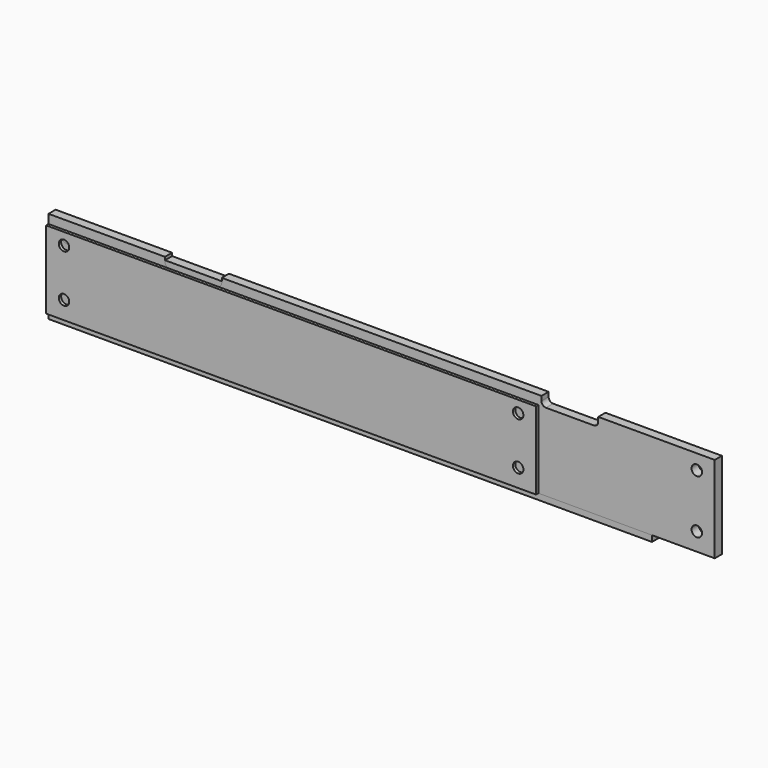
from build123d import *

# Parameters (mm, degrees)
F31_DEPTH       = 19.05
F1_DEPTH        = 25.4
F2_R            = 7.9375
F3_DEPTH        = 50.8
F4_W            = 996.95
F4_H            = 177.8
F5_DEPTH        = 19.05
F6_R            = 3.175
F7_DEPTH        = 25.4
F8_W            = 1041.4
F8_H            = 165.1
F9_DEPTH        = 25.4
F10_R           = 11.1125
F11_DEPTH       = 25.4
F12_R           = 3.96875
F13_DEPTH       = 38.1
F14_R           = 11.1125
F15_DEPTH       = 25.4
F16_R           = 3.96875
F17_DEPTH       = 38.1
F18_W           = 1143
F18_H           = 95.25
F19_DEPTH       = 19.05
F21_D           = 6.35
F21_CBORE_D     = 12.7
F21_CBORE_DEPTH = 9.525
F22_W           = 1416.05
F22_H           = 184.15
F23_DEPTH       = 19.05
F24_W           = 120.65
F24_H           = 19.05
F25_DEPTH       = 25.4
F26_D           = 22.225
F28_D           = 6.35
F28_DEPTH       = 38.1
F28_TIP         = 1.9077324654
F29_R           = 9.525


with BuildPart() as f31:
    # F30 (on Front) → F31 (new body)
    with BuildSketch(Plane.XZ):
        Polygon((0, 0), (0, -12.7), (1282.7, -12.7), (1282.7, 0), (1130.3, 152.4), (152.4, 152.4), align=None)
    extrude(amount=F31_DEPTH)

    # F0 (on face) → F1 (cut)
    with BuildSketch(Plane.XZ.offset(19.05)):
        with BuildLine():
            ThreePointArc((123.825, 111.125), (123.611140622, 117.0632192174), (122.9706705639, 122.9706705639))
            Line((122.9706705639, 122.9706705639), (29.4293294361, 29.4293294361))
            ThreePointArc((29.4293294361, 29.4293294361), (95.2964882938, 48.7056015527), (123.825, 111.125))
        make_face()
        with BuildLine():
            Line((29.4293294361, 29.4293294361), (122.9706705639, 122.9706705639))
            ThreePointArc((122.9706705639, 122.9706705639), (-17.0966647869, 169.496664787), (29.4293294361, 29.4293294361))
        make_face()
        with BuildLine():
            Line((1253.2706705639, 29.4293294361), (1159.7293294361, 122.9706705639))
            ThreePointArc((1159.7293294361, 122.9706705639), (1183.0533352131, 52.7533352131), (1253.2706705639, 29.4293294361))
        make_face()
        with BuildLine():
            ThreePointArc((1253.2706705639, 29.4293294361), (1303.8443984473, 57.1035117062), (1323.975, 111.125))
            ThreePointArc((1323.975, 111.125), (1247.3632192174, 193.461140622), (1159.7293294361, 122.9706705639))
            Line((1159.7293294361, 122.9706705639), (1253.2706705639, 29.4293294361))
        make_face()
    extrude(amount=-F1_DEPTH, mode=Mode.SUBTRACT)

    # F2 (on face) → F3 (cut)
    with BuildSketch(Plane.XZ.offset(19.05)):
        with Locations((361.95, 130.175)):
            Circle(F2_R)
        with Locations((641.35, 130.175)):
            Circle(F2_R)
        with Locations((920.75, 130.175)):
            Circle(F2_R)
    extrude(amount=-F3_DEPTH, mode=Mode.SUBTRACT)


with BuildPart() as f5:
    # F4 (on Front) → F5 (new body)
    with BuildSketch(Plane.XZ):
        with Locations((498.475, 88.9)):
            Rectangle(F4_W, F4_H)
    extrude(amount=F5_DEPTH)

    # F6 (on face) → F7 (cut)
    with BuildSketch(Plane.XZ.offset(19.05)):
        with Locations((958.85, 152.4)):
            Circle(F6_R)
        with Locations((958.85, 41.275)):
            Circle(F6_R)
        with Locations((492.125, 139.7)):
            Circle(F6_R)
        with Locations((492.125, 25.4)):
            Circle(F6_R)
        with Locations((38.1, 152.4)):
            Circle(F6_R)
        with Locations((38.1, 41.275)):
            Circle(F6_R)
        with Locations((101.6, 152.4)):
            Circle(F6_R)
        with Locations((101.6, 41.275)):
            Circle(F6_R)
        with Locations((895.35, 152.4)):
            Circle(F6_R)
        with Locations((895.35, 41.275)):
            Circle(F6_R)
    extrude(amount=-F7_DEPTH, mode=Mode.SUBTRACT)


with BuildPart() as f9:
    # F8 (on Front) → F9 (new body)
    with BuildSketch(Plane.XZ):
        with Locations((520.7, 82.55)):
            Rectangle(F8_W, F8_H)
    extrude(amount=F9_DEPTH)

    # F10 (on face) → F11 (cut)
    with BuildSketch(Plane.XZ.offset(25.4)):
        with Locations((1003.3, 139.7)):
            Circle(F10_R)
        with Locations((1003.3, 38.1)):
            Circle(F10_R)
    extrude(amount=-F11_DEPTH, mode=Mode.SUBTRACT)

    # F12 (on face) → F13 (cut)
    with BuildSketch(Plane.YZ.offset(1041.4)):
        with Locations((-12.7, 38.1)):
            Circle(F12_R)
        with Locations((-12.7, 139.7)):
            Circle(F12_R)
    extrude(amount=-F13_DEPTH, mode=Mode.SUBTRACT)

    # F14 (on face) → F15 (cut)
    with BuildSketch(Plane.XZ.offset(25.4)):
        with Locations((38.1, 139.7)):
            Circle(F14_R)
        with Locations((38.1, 38.1)):
            Circle(F14_R)
    extrude(amount=-F15_DEPTH, mode=Mode.SUBTRACT)

    # F16 (on face) → F17 (cut)
    with BuildSketch(Plane(origin=(0, 0, 0), x_dir=(0, -1, 0), z_dir=(-1, 0, 0))):
        with Locations((12.7, 139.7)):
            Circle(F16_R)
        with Locations((12.7, 38.1)):
            Circle(F16_R)
    extrude(amount=-F17_DEPTH, mode=Mode.SUBTRACT)


with BuildPart() as f19:
    # F18 (on Front) → F19 (new body)
    with BuildSketch(Plane.XZ):
        with Locations((571.5, 47.625)):
            Rectangle(F18_W, F18_H)
    extrude(amount=F19_DEPTH)

    # F21 (through all)
    with Locations(Plane.XZ.offset(19.05)):
        with Locations((19.05, 76.2), (38.1, 76.2), (19.05, 19.05), (38.1, 19.05), (571.5, 76.2), (571.5, 19.05), (1104.9, 76.2), (1125.5375, 76.2), (1104.9, 19.05), (1123.95, 19.05)):
            CounterBoreHole(F21_D / 2, F21_CBORE_D / 2, F21_CBORE_DEPTH)


with BuildPart() as f23:
    # F22 (on Front) → F23 (new body)
    with BuildSketch(Plane.XZ):
        with Locations((708.025, 92.075)):
            Rectangle(F22_W, F22_H)
    extrude(amount=F23_DEPTH)

    # F24 (on face) → F25 (cut)
    with BuildSketch(Plane.XZ.offset(19.05)):
        with Locations((307.975, 174.625)):
            Rectangle(F24_W, F24_H)
        with Locations((1108.075, 174.625)):
            Rectangle(F24_W, F24_H)
    extrude(amount=-F25_DEPTH, mode=Mode.SUBTRACT)

    # F26 (through all)
    with Locations(Plane.XZ.offset(19.05)):
        with Locations((38.1, 152.4), (38.1, 38.1), (1377.95, 152.4), (1377.95, 38.1), (457.2, 41.275), (958.85, 41.275)):
            Hole(F26_D / 2)

    # F28
    with Locations(Plane(origin=(0, 0, 0), x_dir=(0, -1, 0), z_dir=(-1, 0, 0))):
        with Locations((9.525, 152.4), (9.525, 38.1)):
            Hole(F28_D / 2, depth=F28_DEPTH)
            with Locations((0, 0, -(F28_DEPTH + F28_TIP / 2))):  # 118° drill point
                Cone(0, F28_D / 2, F28_TIP, mode=Mode.SUBTRACT)

    # F29
    f29_edges = [f23.edges().sort_by_distance(p)[0] for p in [
        (368.3, -9.525, 165.1),
        (247.65, -9.525, 165.1),
        (1168.4, -9.525, 165.1),
        (1047.75, -9.525, 165.1),
    ]]
    fillet(f29_edges, radius=F29_R)


solid = Compound([f31.part, f5.part, f9.part, f19.part, f23.part])
